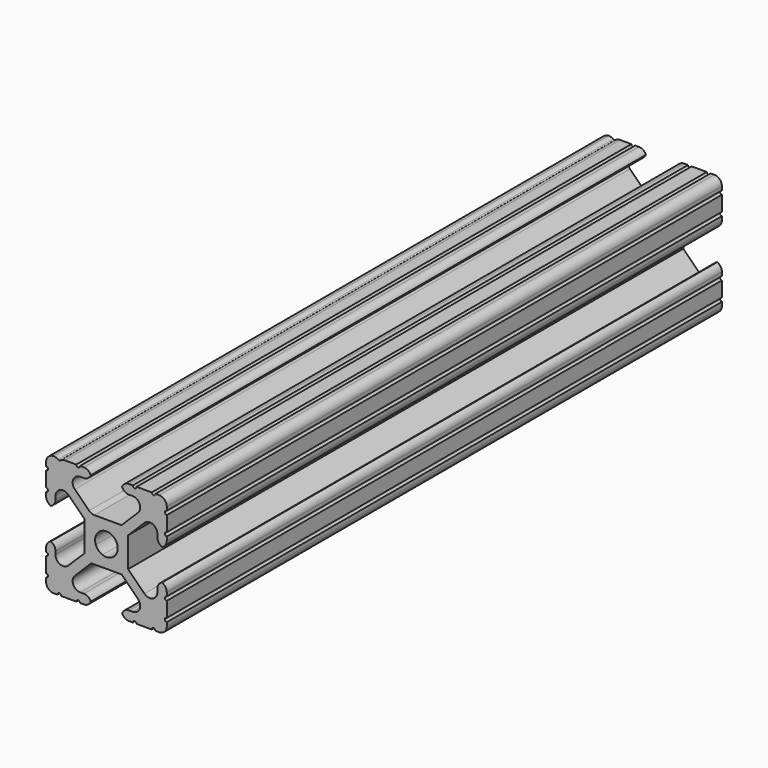
from build123d import *

# Parameters (mm, degrees)
F1_DEPTH    = 146.05
F2_T1_DEPTH = 146.05
F2_T3_DEPTH = 153.9875
F2_T5_DEPTH = 150.01875


# Not quite as in the source:
# - a fillet or chamfer that OpenCascade refuses, or shapes differently, is made with other operations: its cross-section is extruded or revolved along the edge and cut away or added


with BuildPart() as f1:
    # F0 (on Front) → F1 (new body)
    with BuildSketch(Plane.XZ):
        with BuildLine():
            ThreePointArc((-0.8361427067, 2.2296225996), (0, 2.38125), (0.8361427067, 2.2296225996))
            Line((0.8361427067, 2.2296225996), (3.1853789104, 4.5640625))
            Line((3.1853789104, 4.5640625), (-3.1853789104, 4.5640625))
            Line((-3.1853789104, 4.5640625), (-0.8361427067, 2.2296225996))
        make_face()
        with BuildLine():
            ThreePointArc((-2.2347427098, 0.8223603732), (-1.6889881746, 1.6785918231), (-0.8361427067, 2.2296225996))
            Line((-0.8361427067, 2.2296225996), (-3.1853789104, 4.5640625))
            Line((-3.1853789104, 4.5640625), (-4.5640625, 4.5640625))
            Line((-4.5640625, 4.5640625), (-4.5640625, 3.1376763557))
            Line((-4.5640625, 3.1376763557), (-2.2347427098, 0.8223603732))
        make_face()
        with BuildLine():
            ThreePointArc((-2.2347427098, -0.8223603732), (-2.38125, 0), (-2.2347427098, 0.8223603732))
            Line((-2.2347427098, 0.8223603732), (-4.5640625, 3.1376763557))
            Line((-4.5640625, 3.1376763557), (-4.5640625, -3.1376763557))
            Line((-4.5640625, -3.1376763557), (-2.2347427098, -0.8223603732))
        make_face()
        with BuildLine():
            Line((-3.1853789104, -4.5640625), (-0.8361427067, -2.2296225996))
            ThreePointArc((-0.8361427067, -2.2296225996), (-1.6889881746, -1.6785918231), (-2.2347427098, -0.8223603732))
            Line((-2.2347427098, -0.8223603732), (-4.5640625, -3.1376763557))
            Line((-4.5640625, -3.1376763557), (-4.5640625, -4.5640625))
            Line((-4.5640625, -4.5640625), (-3.1853789104, -4.5640625))
        make_face()
        with BuildLine():
            Line((3.1853789104, -4.5640625), (0.8361427067, -2.2296225996))
            ThreePointArc((0.8361427067, -2.2296225996), (0, -2.38125), (-0.8361427067, -2.2296225996))
            Line((-0.8361427067, -2.2296225996), (-3.1853789104, -4.5640625))
            Line((-3.1853789104, -4.5640625), (3.1853789104, -4.5640625))
        make_face()
        with BuildLine():
            Line((4.5640625, -3.1376763557), (2.2347427098, -0.8223603732))
            ThreePointArc((2.2347427098, -0.8223603732), (1.6889881746, -1.6785918231), (0.8361427067, -2.2296225996))
            Line((0.8361427067, -2.2296225996), (3.1853789104, -4.5640625))
            Line((3.1853789104, -4.5640625), (4.5640625, -4.5640625))
            Line((4.5640625, -4.5640625), (4.5640625, -3.1376763557))
        make_face()
        with BuildLine():
            ThreePointArc((2.2347427098, 0.8223603732), (2.3443370748, 0.4176544533), (2.38125, 0))
            ThreePointArc((2.38125, 0), (2.3443370748, -0.4176544533), (2.2347427098, -0.8223603732))
            Line((2.2347427098, -0.8223603732), (4.5640625, -3.1376763557))
            Line((4.5640625, -3.1376763557), (4.5640625, 3.1376763557))
            Line((4.5640625, 3.1376763557), (2.2347427098, 0.8223603732))
        make_face()
        with BuildLine():
            ThreePointArc((0.8361427067, 2.2296225996), (1.6889881746, 1.6785918231), (2.2347427098, 0.8223603732))
            Line((2.2347427098, 0.8223603732), (4.5640625, 3.1376763557))
            Line((4.5640625, 3.1376763557), (4.5640625, 4.5640625))
            Line((4.5640625, 4.5640625), (3.1853789104, 4.5640625))
            Line((3.1853789104, 4.5640625), (0.8361427067, 2.2296225996))
        make_face()
        Polygon((4.5640625, 4.5640625), (4.5640625, 3.1376763557), (10.715625, 9.2522558281), (12.7, 11.2247008192), (12.7, 12.7), (11.3728841543, 12.7), (9.3759316558, 10.715625), (3.1853789104, 4.5640625), align=None)
        with BuildLine():
            Line((12.7, 11.2247008192), (10.715625, 9.2522558281))
            Line((10.715625, 9.2522558281), (10.715625, 7.14375))
            Line((10.715625, 7.14375), (10.715625, 3.175))
            Line((10.715625, 3.175), (12.7, 3.175))
            Line((12.7, 3.175), (12.7, 5.55625))
            ThreePointArc((12.7, 5.55625), (12.303125, 5.953125), (12.7, 6.35))
            Line((12.7, 6.35), (12.7, 9.525))
            ThreePointArc((12.7, 9.525), (12.303125, 9.921875), (12.7, 10.31875))
            Line((12.7, 10.31875), (12.7, 11.2247008192))
        make_face()
        with BuildLine():
            Line((7.14375, 10.715625), (9.3759316558, 10.715625))
            Line((9.3759316558, 10.715625), (11.3728841543, 12.7))
            Line((11.3728841543, 12.7), (10.31875, 12.7))
            ThreePointArc((10.31875, 12.7), (9.921875, 12.303125), (9.525, 12.7))
            Line((9.525, 12.7), (6.35, 12.7))
            ThreePointArc((6.35, 12.7), (5.953125, 12.303125), (5.55625, 12.7))
            Line((5.55625, 12.7), (3.175, 12.7))
            Line((3.175, 12.7), (3.175, 10.715625))
            Line((3.175, 10.715625), (7.14375, 10.715625))
        make_face()
        with BuildLine():
            Line((-11.3728841543, 12.7), (-9.3759316558, 10.715625))
            Line((-9.3759316558, 10.715625), (-7.14375, 10.715625))
            Line((-7.14375, 10.715625), (-3.175, 10.715625))
            Line((-3.175, 10.715625), (-3.175, 12.7))
            Line((-3.175, 12.7), (-5.55625, 12.7))
            ThreePointArc((-5.55625, 12.7), (-5.953125, 12.303125), (-6.35, 12.7))
            Line((-6.35, 12.7), (-7.14375, 12.7))
            Line((-7.14375, 12.7), (-9.525, 12.7))
            ThreePointArc((-9.525, 12.7), (-9.921875, 12.303125), (-10.31875, 12.7))
            Line((-10.31875, 12.7), (-11.3728841543, 12.7))
        make_face()
        Polygon((-4.5640625, 4.5640625), (-3.1853789104, 4.5640625), (-9.3759316558, 10.715625), (-11.3728841543, 12.7), (-12.7, 11.2247008192), (-10.715625, 9.2522558281), (-4.5640625, 3.1376763557), align=None)
        Polygon((-12.7, 11.2247008192), (-11.3728841543, 12.7), (-12.7, 12.7), align=None)
        with BuildLine():
            Line((-10.715625, 7.14375), (-10.715625, 9.2522558281))
            Line((-10.715625, 9.2522558281), (-12.7, 11.2247008192))
            Line((-12.7, 11.2247008192), (-12.7, 10.31875))
            ThreePointArc((-12.7, 10.31875), (-12.303125, 9.921875), (-12.7, 9.525))
            Line((-12.7, 9.525), (-12.7, 6.35))
            ThreePointArc((-12.7, 6.35), (-12.303125, 5.953125), (-12.7, 5.55625))
            Line((-12.7, 5.55625), (-12.7, 3.175))
            Line((-12.7, 3.175), (-10.715625, 3.175))
            Line((-10.715625, 3.175), (-10.715625, 7.14375))
        make_face()
        with BuildLine():
            Line((-12.7, -11.2247008192), (-10.715625, -9.2522558281))
            Line((-10.715625, -9.2522558281), (-10.715625, -7.14375))
            Line((-10.715625, -7.14375), (-10.715625, -3.175))
            Line((-10.715625, -3.175), (-12.7, -3.175))
            Line((-12.7, -3.175), (-12.7, -5.55625))
            ThreePointArc((-12.7, -5.55625), (-12.303125, -5.953125), (-12.7, -6.35))
            Line((-12.7, -6.35), (-12.7, -9.525))
            ThreePointArc((-12.7, -9.525), (-12.303125, -9.921875), (-12.7, -10.31875))
            Line((-12.7, -10.31875), (-12.7, -11.2247008192))
        make_face()
        Polygon((-9.3759316558, -10.715625), (-3.1853789104, -4.5640625), (-4.5640625, -4.5640625), (-4.5640625, -3.1376763557), (-10.715625, -9.2522558281), (-12.7, -11.2247008192), (-12.7, -12.7), (-11.3728841543, -12.7), align=None)
        with BuildLine():
            Line((-7.14375, -10.715625), (-9.3759316558, -10.715625))
            Line((-9.3759316558, -10.715625), (-11.3728841543, -12.7))
            Line((-11.3728841543, -12.7), (-10.31875, -12.7))
            ThreePointArc((-10.31875, -12.7), (-9.921875, -12.303125), (-9.525, -12.7))
            Line((-9.525, -12.7), (-6.35, -12.7))
            ThreePointArc((-6.35, -12.7), (-5.953125, -12.303125), (-5.55625, -12.7))
            Line((-5.55625, -12.7), (-3.175, -12.7))
            Line((-3.175, -12.7), (-3.175, -10.715625))
            Line((-3.175, -10.715625), (-7.14375, -10.715625))
        make_face()
        with BuildLine():
            Line((11.3728841543, -12.7), (9.3759316558, -10.715625))
            Line((9.3759316558, -10.715625), (7.14375, -10.715625))
            Line((7.14375, -10.715625), (3.175, -10.715625))
            Line((3.175, -10.715625), (3.175, -12.7))
            Line((3.175, -12.7), (5.55625, -12.7))
            ThreePointArc((5.55625, -12.7), (5.953125, -12.303125), (6.35, -12.7))
            Line((6.35, -12.7), (9.525, -12.7))
            ThreePointArc((9.525, -12.7), (9.921875, -12.303125), (10.31875, -12.7))
            Line((10.31875, -12.7), (11.3728841543, -12.7))
        make_face()
        Polygon((10.715625, -9.2522558281), (4.5640625, -3.1376763557), (4.5640625, -4.5640625), (3.1853789104, -4.5640625), (9.3759316558, -10.715625), (11.3728841543, -12.7), (12.7, -12.7), (12.7, -11.2247008192), align=None)
        with BuildLine():
            Line((10.715625, -7.14375), (10.715625, -9.2522558281))
            Line((10.715625, -9.2522558281), (12.7, -11.2247008192))
            Line((12.7, -11.2247008192), (12.7, -10.31875))
            ThreePointArc((12.7, -10.31875), (12.303125, -9.921875), (12.7, -9.525))
            Line((12.7, -9.525), (12.7, -6.35))
            ThreePointArc((12.7, -6.35), (12.303125, -5.953125), (12.7, -5.55625))
            Line((12.7, -5.55625), (12.7, -3.175))
            Line((12.7, -3.175), (10.715625, -3.175))
            Line((10.715625, -3.175), (10.715625, -7.14375))
        make_face()
    extrude(amount=F1_DEPTH)

    # F2: fillet of radius 1.5875 on 31 edges, made by hand

    # F2_s2 → F2_t1 (join)
    with BuildSketch(Plane.XZ):
        with BuildLine():
            ThreePointArc((-6.6451596968, 8.0020523886), (-6.9937960043, 9.7333175229), (-5.5261794807, 10.715625))
            Line((-5.5261794807, 10.715625), (-9.3759316558, 10.715625))
            Line((-9.3759316558, 10.715625), (-6.6451596968, 8.0020523886))
        make_face()
        with BuildLine():
            ThreePointArc((-8.0089825615, 6.5618856508), (-9.7378452755, 6.9017155215), (-10.715625, 5.4359742634))
            Line((-10.715625, 5.4359742634), (-10.715625, 9.2522558281))
            Line((-10.715625, 9.2522558281), (-8.0089825615, 6.5618856508))
        make_face()
        with BuildLine():
            ThreePointArc((5.5261794807, 10.715625), (6.9937960043, 9.7333175229), (6.6451596968, 8.0020523886))
            Line((6.6451596968, 8.0020523886), (9.3759316558, 10.715625))
            Line((9.3759316558, 10.715625), (5.5261794807, 10.715625))
        make_face()
        with BuildLine():
            ThreePointArc((8.0089825615, 6.5618856508), (9.7378452755, 6.9017155215), (10.715625, 5.4359742634))
            Line((10.715625, 5.4359742634), (10.715625, 9.2522558281))
            Line((10.715625, 9.2522558281), (8.0089825615, 6.5618856508))
        make_face()
        with BuildLine():
            ThreePointArc((10.715625, -5.4359742634), (9.7378452755, -6.9017155215), (8.0089825615, -6.5618856508))
            Line((8.0089825615, -6.5618856508), (10.715625, -9.2522558281))
            Line((10.715625, -9.2522558281), (10.715625, -5.4359742634))
        make_face()
        with BuildLine():
            ThreePointArc((6.6451596968, -8.0020523886), (6.9937960043, -9.7333175229), (5.5261794807, -10.715625))
            Line((5.5261794807, -10.715625), (9.3759316558, -10.715625))
            Line((9.3759316558, -10.715625), (6.6451596968, -8.0020523886))
        make_face()
        with BuildLine():
            ThreePointArc((-5.5261794807, -10.715625), (-6.9937960043, -9.7333175229), (-6.6451596968, -8.0020523886))
            Line((-6.6451596968, -8.0020523886), (-9.3759316558, -10.715625))
            Line((-9.3759316558, -10.715625), (-5.5261794807, -10.715625))
        make_face()
        with BuildLine():
            ThreePointArc((-8.0089825615, -6.5618856508), (-9.7378452755, -6.9017155215), (-10.715625, -5.4359742634))
            Line((-10.715625, -5.4359742634), (-10.715625, -9.2522558281))
            Line((-10.715625, -9.2522558281), (-8.0089825615, -6.5618856508))
        make_face()
        with BuildLine():
            ThreePointArc((-2.530750733, 4.5640625), (-3.1359432558, 4.6839459764), (-3.649730949, 5.0254898886))
            Line((-3.649730949, 5.0254898886), (-3.1853789104, 4.5640625))
            Line((-3.1853789104, 4.5640625), (-2.530750733, 4.5640625))
        make_face()
    extrude(amount=F2_T1_DEPTH)

    # F2_s4 → F2_t3 (cut)
    with BuildSketch(Plane.XZ.offset(-3.96875)):
        with BuildLine():
            ThreePointArc((-12.7, -11.1125), (-12.2350320151, -12.2350320151), (-11.1125, -12.7))
            Line((-11.1125, -12.7), (-12.7, -12.7))
            Line((-12.7, -12.7), (-12.7, -11.1125))
        make_face()
        with BuildLine():
            ThreePointArc((11.1125, -12.7), (12.2350320151, -12.2350320151), (12.7, -11.1125))
            Line((12.7, -11.1125), (12.7, -12.7))
            Line((12.7, -12.7), (11.1125, -12.7))
        make_face()
        with BuildLine():
            ThreePointArc((12.7, 11.1125), (12.2350320151, 12.2350320151), (11.1125, 12.7))
            Line((11.1125, 12.7), (12.7, 12.7))
            Line((12.7, 12.7), (12.7, 11.1125))
        make_face()
        with BuildLine():
            ThreePointArc((-12.7, 4.7625), (-12.2350320151, 3.6399679849), (-11.1125, 3.175))
            Line((-11.1125, 3.175), (-12.7, 3.175))
            Line((-12.7, 3.175), (-12.7, 4.7625))
        make_face()
        with BuildLine():
            ThreePointArc((-11.1125, -3.175), (-12.2350320151, -3.6399679849), (-12.7, -4.7625))
            Line((-12.7, -4.7625), (-12.7, -3.175))
            Line((-12.7, -3.175), (-11.1125, -3.175))
        make_face()
        with BuildLine():
            ThreePointArc((-12.303125, 3.175), (-11.1805929849, 3.6399679849), (-10.715625, 4.7625))
            Line((-10.715625, 4.7625), (-10.715625, 3.175))
            Line((-10.715625, 3.175), (-12.303125, 3.175))
        make_face()
        with BuildLine():
            ThreePointArc((-10.715625, -4.7625), (-11.1805929849, -3.6399679849), (-12.303125, -3.175))
            Line((-12.303125, -3.175), (-10.715625, -3.175))
            Line((-10.715625, -3.175), (-10.715625, -4.7625))
        make_face()
        with BuildLine():
            ThreePointArc((-3.175, -12.303125), (-3.6399679849, -11.1805929849), (-4.7625, -10.715625))
            Line((-4.7625, -10.715625), (-3.175, -10.715625))
            Line((-3.175, -10.715625), (-3.175, -12.303125))
        make_face()
        with BuildLine():
            ThreePointArc((-4.7625, -12.7), (-3.6399679849, -12.2350320151), (-3.175, -11.1125))
            Line((-3.175, -11.1125), (-3.175, -12.7))
            Line((-3.175, -12.7), (-4.7625, -12.7))
        make_face()
        with BuildLine():
            ThreePointArc((3.175, -11.1125), (3.6399679849, -12.2350320151), (4.7625, -12.7))
            Line((4.7625, -12.7), (3.175, -12.7))
            Line((3.175, -12.7), (3.175, -11.1125))
        make_face()
        with BuildLine():
            ThreePointArc((4.7625, -10.715625), (3.6399679849, -11.1805929849), (3.175, -12.303125))
            Line((3.175, -12.303125), (3.175, -10.715625))
            Line((3.175, -10.715625), (4.7625, -10.715625))
        make_face()
        with BuildLine():
            ThreePointArc((12.7, -4.7625), (12.2350320151, -3.6399679849), (11.1125, -3.175))
            Line((11.1125, -3.175), (12.7, -3.175))
            Line((12.7, -3.175), (12.7, -4.7625))
        make_face()
        with BuildLine():
            ThreePointArc((11.1125, 3.175), (12.2350320151, 3.6399679849), (12.7, 4.7625))
            Line((12.7, 4.7625), (12.7, 3.175))
            Line((12.7, 3.175), (11.1125, 3.175))
        make_face()
        with BuildLine():
            ThreePointArc((12.303125, -3.175), (11.1805929849, -3.6399679849), (10.715625, -4.7625))
            Line((10.715625, -4.7625), (10.715625, -3.175))
            Line((10.715625, -3.175), (12.303125, -3.175))
        make_face()
        with BuildLine():
            ThreePointArc((10.715625, 4.7625), (11.1805929849, 3.6399679849), (12.303125, 3.175))
            Line((12.303125, 3.175), (10.715625, 3.175))
            Line((10.715625, 3.175), (10.715625, 4.7625))
        make_face()
        with BuildLine():
            ThreePointArc((-4.7625, 10.715625), (-3.6399679849, 11.1805929849), (-3.175, 12.303125))
            Line((-3.175, 12.303125), (-3.175, 10.715625))
            Line((-3.175, 10.715625), (-4.7625, 10.715625))
        make_face()
        with BuildLine():
            ThreePointArc((-3.175, 11.1125), (-3.6399679849, 12.2350320151), (-4.7625, 12.7))
            Line((-4.7625, 12.7), (-3.175, 12.7))
            Line((-3.175, 12.7), (-3.175, 11.1125))
        make_face()
        with BuildLine():
            ThreePointArc((4.7625, 12.7), (3.6399679849, 12.2350320151), (3.175, 11.1125))
            Line((3.175, 11.1125), (3.175, 12.7))
            Line((3.175, 12.7), (4.7625, 12.7))
        make_face()
        with BuildLine():
            ThreePointArc((3.175, 12.303125), (3.6399679849, 11.1805929849), (4.7625, 10.715625))
            Line((4.7625, 10.715625), (3.175, 10.715625))
            Line((3.175, 10.715625), (3.175, 12.303125))
        make_face()
        with BuildLine():
            ThreePointArc((-11.1125, 12.7), (-12.2350320151, 12.2350320151), (-12.7, 11.1125))
            Line((-12.7, 11.1125), (-12.7, 12.7))
            Line((-12.7, 12.7), (-11.1125, 12.7))
        make_face()
    extrude(amount=F2_T3_DEPTH, mode=Mode.SUBTRACT)

    # F2_s6 → F2_t5 (cut)
    with BuildSketch(Plane.XZ.offset(-1.984375)):
        with BuildLine():
            ThreePointArc((-8.73125, 12.7), (-9.2332615786, 12.6185347357), (-9.68375, 12.3825))
            ThreePointArc((-9.68375, 12.3825), (-9.5668992086, 12.5225121043), (-9.525, 12.7))
            Line((-9.525, 12.7), (-8.73125, 12.7))
        make_face()
        with BuildLine():
            ThreePointArc((-10.16, 12.3825), (-10.6104884214, 12.6185347357), (-11.1125, 12.7))
            Line((-11.1125, 12.7), (-10.31875, 12.7))
            ThreePointArc((-10.31875, 12.7), (-10.2768507914, 12.5225121043), (-10.16, 12.3825))
        make_face()
    extrude(amount=F2_T5_DEPTH, mode=Mode.SUBTRACT)


solid = f1.part
